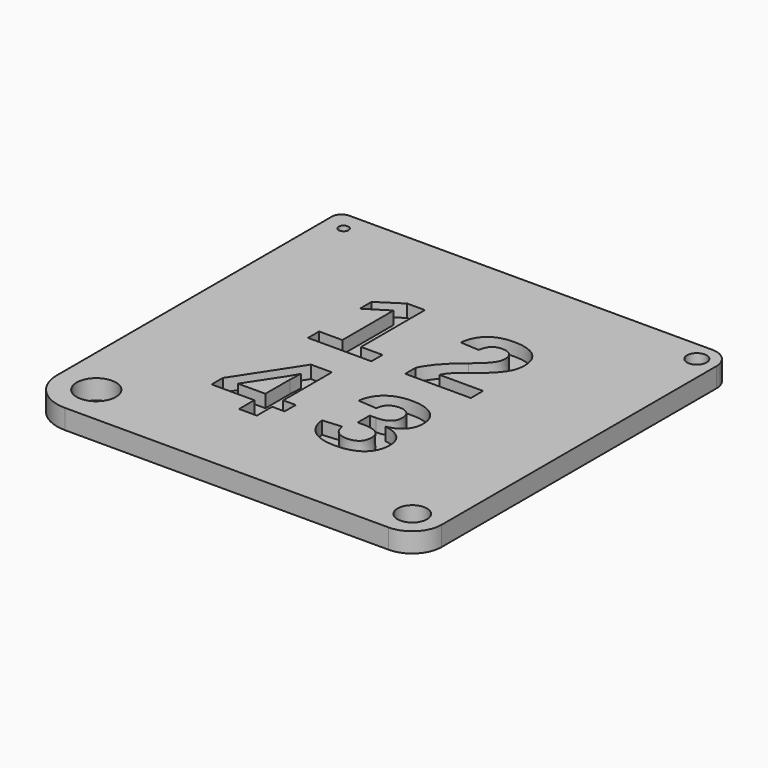
from build123d import *

# Parameters (mm, degrees)
F1_DEPTH     = 2
F2_R         = 0.5
F2_R_2       = 1
F2_R_3       = 1.5
F2_R_4       = 2
F3_DEPTH     = 25
F2_TEXT_SIZE = 13.8888888889
F4_DEPTH     = 1.3


# Not quite as in the source:
# - Text() gives the source's letters only with a copy of the font that has no kerning and outlines rounded to 1/6400 em; it was checked with that copy


with BuildPart() as f1:
    # F0 (on Top) → F1 (new body)
    with BuildSketch(Plane.XY):
        with BuildLine():
            Line((18, 20), (-19, 20))
            ThreePointArc((-19, 20), (-19.7071067812, 19.7071067812), (-20, 19))
            Line((-20, 19), (-20, -16))
            ThreePointArc((-20, -16), (-18.8284271247, -18.8284271247), (-16, -20))
            Line((-16, -20), (17, -20))
            ThreePointArc((17, -20), (19.1213203436, -19.1213203436), (20, -17))
            Line((20, -17), (20, 18))
            ThreePointArc((20, 18), (19.4142135624, 19.4142135624), (18, 20))
        make_face()
    extrude(amount=F1_DEPTH)

    # F2 (on face) → F3 (cut)
    with BuildSketch(Plane.XY.offset(2)):
        with Locations((-18, 18)):
            Circle(F2_R)
        with Locations((18, 18)):
            Circle(F2_R_2)
        with Locations((17, -17)):
            Circle(F2_R_3)
        with Locations((-16, -16)):
            Circle(F2_R_4)
    extrude(amount=-F3_DEPTH, mode=Mode.SUBTRACT)

    # F2 (on face) → F4 (cut)
    with BuildSketch(Plane.XY.offset(2)):
        with Locations((-9.30078125, 1.5)):
            Text('1', F2_TEXT_SIZE, font='Arimo', font_style=FontStyle.BOLD, text_align=(TextAlign.LEFT, TextAlign.BOTTOM))
        with Locations((1, 1.5)):
            Text('2', F2_TEXT_SIZE, font='Arimo', font_style=FontStyle.BOLD, text_align=(TextAlign.LEFT, TextAlign.BOTTOM))
        with Locations((1, -11.5)):
            Text('3', F2_TEXT_SIZE, font='Arimo', font_style=FontStyle.BOLD, text_align=(TextAlign.LEFT, TextAlign.BOTTOM))
        with Locations((-9.61328125, -11.5)):
            Text('4', F2_TEXT_SIZE, font='Arimo', font_style=FontStyle.BOLD, text_align=(TextAlign.LEFT, TextAlign.BOTTOM))
    extrude(amount=-F4_DEPTH, mode=Mode.SUBTRACT)


solid = f1.part
